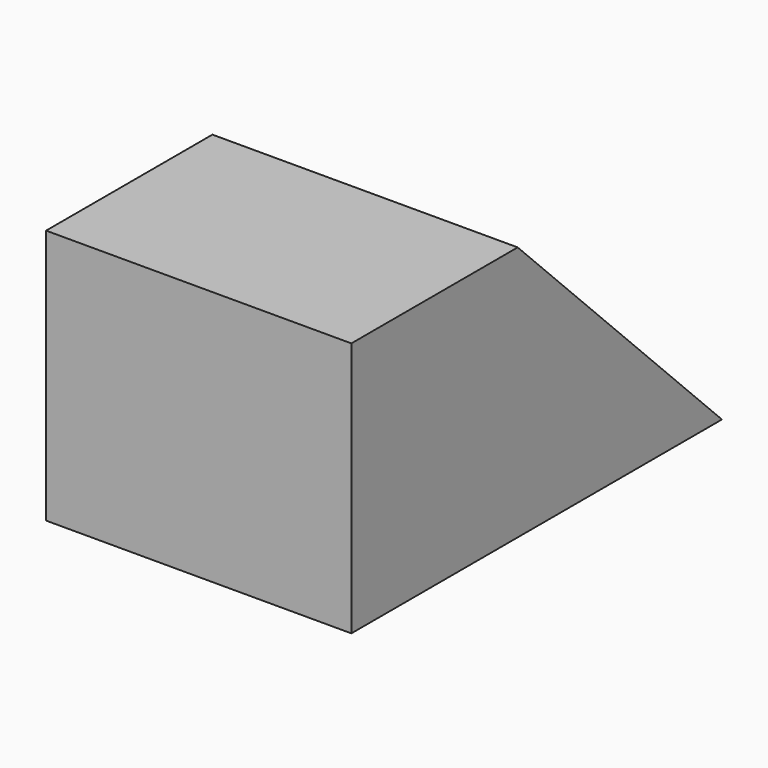
from build123d import *

# Parameters (mm, degrees)
F0_W        = 47.8297565132
F0_H        = 76.5759237111
F1_DEPTH    = 40
F2_T1_DEPTH = 274.1378594542
F3_T        = -2


# Not quite as in the source:
# - a fillet or chamfer that OpenCascade refuses, or shapes differently, is made with other operations: its cross-section is extruded or revolved along the edge and cut away or added


with BuildPart() as f1:
    # F0 (on Top) → F1 (new body)
    with BuildSketch(Plane.XY):
        with Locations((-40.5828235671, -10.7496175915)):
            Rectangle(F0_W, F0_H)
    extrude(amount=F1_DEPTH)

    # F2: chamfer of 44 on 1 edges, made by hand

    # F2_s2 → F2_t1 (cut)
    with BuildSketch(Plane.YZ.offset(-177.6517532942)):
        Polygon((27.538344264, -4), (-16.461655736, 40), (27.538344264, 40), align=None)
    extrude(amount=F2_T1_DEPTH, mode=Mode.SUBTRACT)

    # F3
    f3_openings = [f1.faces().sort_by_distance(p)[0] for p in [
        (-40.582824, 3.538344, 20),
    ]]
    offset(amount=F3_T, openings=f3_openings, kind=Kind.INTERSECTION)


solid = f1.part
